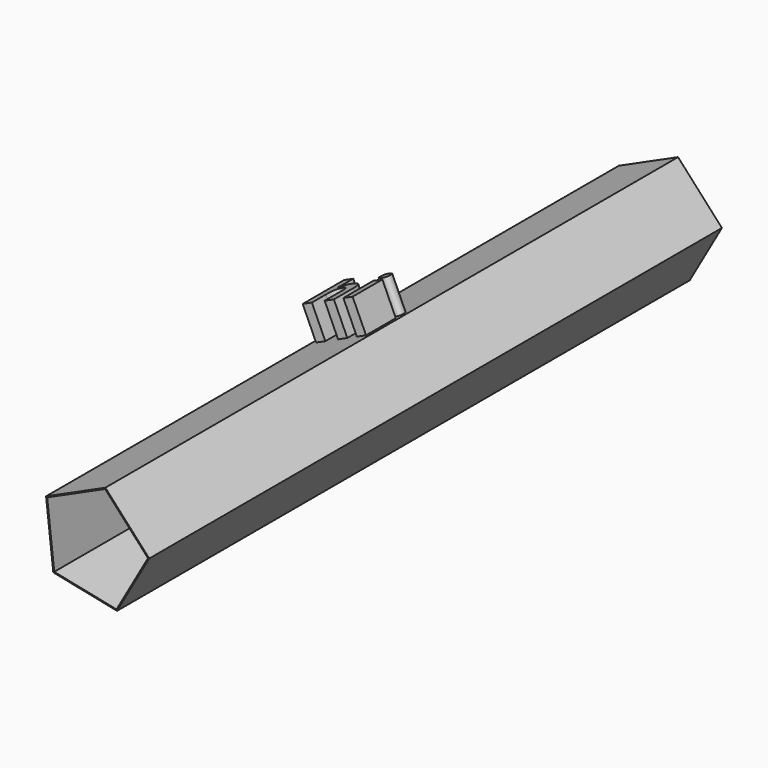
from build123d import *

# Parameters (mm, degrees)
F1_DEPTH     = 440
F2_T         = -0.63
F4_D         = 12.7
F4_DEPTH     = 12.7
F4_TIP       = 3.8154649308
F5_TEXT_SIZE = 41.8437397842
F6_DEPTH     = 20


# Not quite as in the source:
# - Text() gives the source's letters only with a copy of the font that has no kerning and outlines rounded to 1/6400 em; it was checked with that copy


with BuildPart() as f1:
    # F0 (on Front) → F1 (new body)
    with BuildSketch(Plane.XZ):
        Polygon((25.8937657237, 30.8007701662), (-10.5422802089, 14.29578435), (-6.104463298, -25.4572756714), (33.0743043214, -33.5210321052), (52.8502974366, 1.2483523631), align=None)
    extrude(amount=F1_DEPTH)

    # F2
    f2_openings = [f1.faces().sort_by_distance(p)[0] for p in [
        (19.034325, -440, -2.52668),
    ]]
    offset(amount=F2_T, openings=f2_openings)

    # F4
    with Locations(Plane(origin=(-8.8362561265, 0, -0.9864319085), x_dir=(0, -1, 0), z_dir=(-0.9938265005, 0, -0.1109454228))):
        with Locations((198.206230998, 0)):
            Hole(F4_D / 2, depth=F4_DEPTH)
            with Locations((0, 0, -(F4_DEPTH + F4_TIP / 2))):  # 118° drill point
                Cone(0, F4_D / 2, F4_TIP, mode=Mode.SUBTRACT)

    # F5 (on face) → F6 (join)
    with BuildSketch(Plane(origin=(-7.1681363894, 0, 15.8242212168), x_dir=(0.9109011483, 0, 0.4126246454), z_dir=(-0.4126246454, 0, 0.9109011483))):
        with Locations((-3.7041821999, -236.2938960719)):
            Text('hi', F5_TEXT_SIZE, font='Open Sans', font_style=FontStyle.BOLD, text_align=(TextAlign.LEFT, TextAlign.BOTTOM))
    extrude(amount=F6_DEPTH)


solid = f1.part
